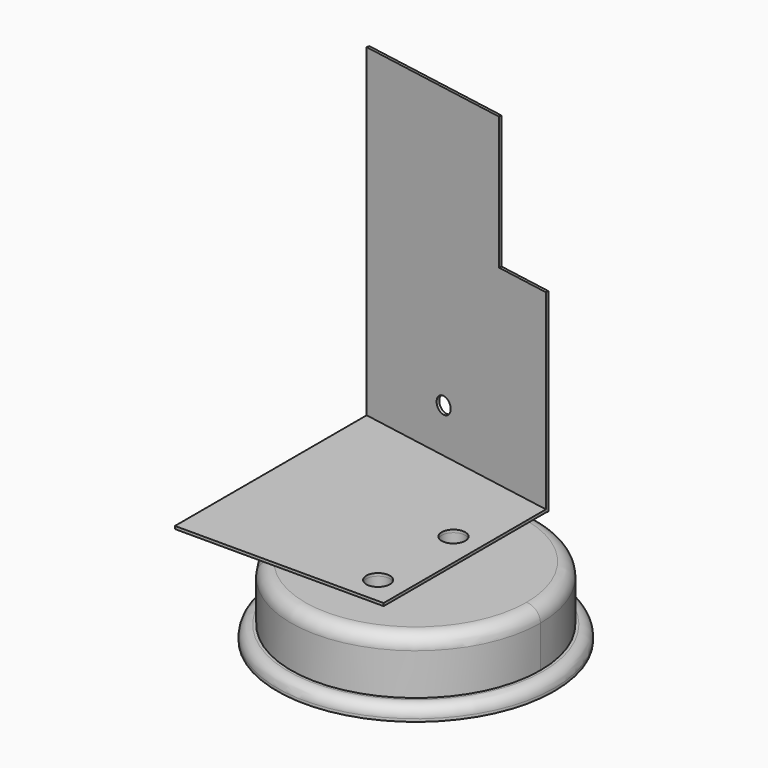
from build123d import *

# Parameters (mm, degrees)
F0_R     = 4.25
F1_DEPTH = 20
F2_R     = 5
F3_R     = 50
F3_R_2   = 45
F3_R_3   = 4.25
F4_DEPTH = 5
F5_R     = 4
F6_R     = 4.25
F7_DEPTH = 1
F8_W     = 76.5163908218
F8_H     = 1
F8_R     = 3
F9_DEPTH = 1


# Not quite as in the source:
# - a feature names something its author has since deleted; it is built from what else it names


with BuildPart() as f1:
    # F0 (on Top) → F1 (new body)
    with BuildSketch(Plane.XY):
        with BuildLine():
            Line((10, -27), (10, 43.874821937))
            ThreePointArc((10, 43.874821937), (-37.7466567546, 24.4987735173), (-36, -27))
            Line((-36, -27), (10, -27))
        make_face()
        with Locations((0, -17)):
            Circle(F0_R, mode=Mode.SUBTRACT)
        with Locations((0, 17)):
            Circle(F0_R, mode=Mode.SUBTRACT)
        with BuildLine():
            ThreePointArc((-36, -27), (14.2302494708, -42.6907484123), (45, 0))
            ThreePointArc((45, 0), (35.1781181987, 28.0624304008), (10, 43.874821937))
            Line((10, 43.874821937), (10, -27))
            Line((10, -27), (-36, -27))
        make_face()
    extrude(amount=-F1_DEPTH)

    # F2
    f2_edges = [f1.edges().sort_by_distance(p)[0] for p in [
        (-10, -43.874822, 0),
    ]]
    fillet(f2_edges, radius=F2_R)


with BuildPart() as f4:
    # F3 (on face) → F4 (new body)
    with BuildSketch(Plane(origin=(0, 0, -20), x_dir=(1, 0, 0), z_dir=(0, 0, -1))):
        Circle(F3_R)
        Circle(F3_R_2, mode=Mode.SUBTRACT)
        Circle(F3_R_2)
        with Locations((0, -17)):
            Circle(F3_R_3, mode=Mode.SUBTRACT)
        with Locations((0, 17)):
            Circle(F3_R_3, mode=Mode.SUBTRACT)
    extrude(amount=F4_DEPTH)

    # F5
    f5_edges = [f4.edges().sort_by_distance(p)[0] for p in [
        (-50, 0, -20),
    ]]
    fillet(f5_edges, radius=F5_R)


with BuildPart() as f7:
    # F6 (on face) → F7 (new body)
    with BuildSketch(Plane.XY):
        with BuildLine():
            Line((10, 46.2367301929), (-65.3539349139, 59.5236620208))
            Line((-65.3539349139, 59.5236620208), (-65.3539349139, -27))
            Line((-65.3539349139, -27), (-29.5127091267, -27))
            ThreePointArc((-29.5127091267, -27), (-34.2824912471, 20.6085126561), (10, 38.7298334621))
            Line((10, 38.7298334621), (10, 46.2367301929))
        make_face()
        with BuildLine():
            ThreePointArc((10, 38.7298334621), (-34.2824912471, 20.6085126561), (-29.5127091267, -27))
            Line((-29.5127091267, -27), (10, -27))
            Line((10, -27), (10, 38.7298334621))
        make_face()
        with Locations((0, -17)):
            Circle(F6_R, mode=Mode.SUBTRACT)
        with Locations((0, 17)):
            Circle(F6_R, mode=Mode.SUBTRACT)
    extrude(amount=F7_DEPTH)

    # F8 (on face) → F9 (join)
    with BuildSketch(Plane(origin=(8.2084834398, 46.5526228989, 0), x_dir=(-0.984807753, 0.1736481777, 0), z_dir=(0.1736481777, 0.984807753, 0))):
        with Locations((36.4390418201, 0.5)):
            Rectangle(F8_W, F8_H)
        Polygon((-1.8191535908, 70), (-1.8191535908, 1), (74.697237231, 1), (74.697237231, 118), (18.1808464092, 118), (18.1808464092, 70), align=None)
        with Locations((41.8441907202, 17)):
            Circle(F8_R, mode=Mode.SUBTRACT)
    extrude(amount=F9_DEPTH)


solid = Compound([f1.part, f4.part, f7.part])
